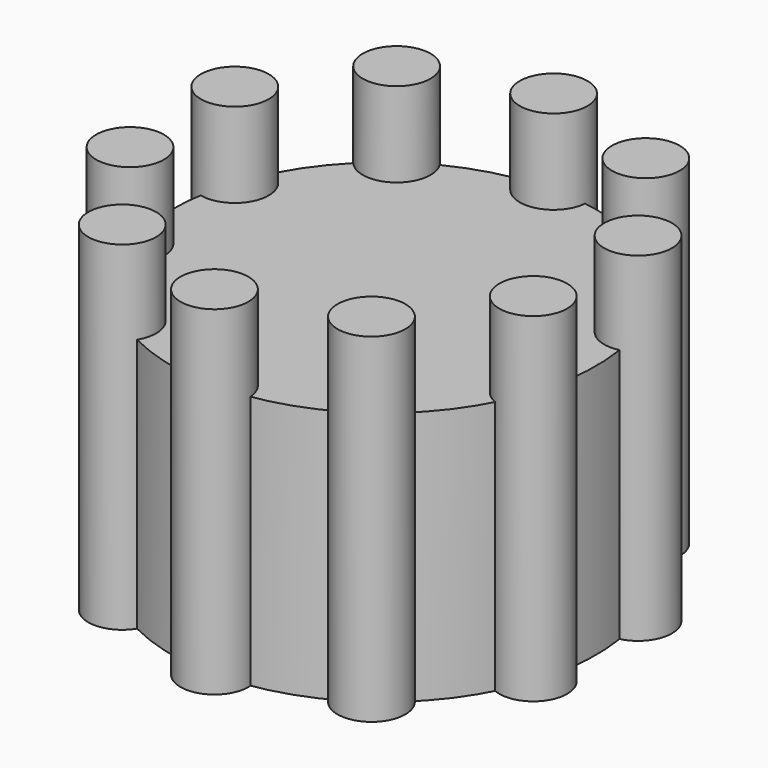
from build123d import *

# Parameters (mm, degrees)
F0_R     = 31.75
F1_DEPTH = 38.1
F2_R     = 5.08
F3_DEPTH = 50.8


with BuildPart() as f1:
    # F0 (on Top) → F1 (new body)
    with BuildSketch(Plane.XY):
        Circle(F0_R)
    extrude(amount=F1_DEPTH)

    # F2 (on Top) → F3, piece 2 (join)
    with BuildSketch(Plane.XY):
        with Locations((-18.6621817603, 25.6862895714)):
            Circle(F2_R)
    extrude(amount=F3_DEPTH)


with BuildPart() as f3:
    # F2 (on Top) → F3 (new body)
    with BuildSketch(Plane.XY):
        with Locations((0, 31.75)):
            Circle(F2_R)
    extrude(amount=F3_DEPTH)


with BuildPart() as f3b:
    # F2 (on Top) → F3, piece 3 (new body)
    with BuildSketch(Plane.XY):
        with Locations((-30.1960443924, 9.8112895714)):
            Circle(F2_R)
    extrude(amount=F3_DEPTH)


with BuildPart() as f3c:
    # F2 (on Top) → F3, piece 4 (new body)
    with BuildSketch(Plane.XY):
        with Locations((-30.1960443924, -9.8112895714)):
            Circle(F2_R)
    extrude(amount=F3_DEPTH)


with BuildPart() as f3d:
    # F2 (on Top) → F3, piece 5 (new body)
    with BuildSketch(Plane.XY):
        with Locations((-18.6621817603, -25.6862895714)):
            Circle(F2_R)
    extrude(amount=F3_DEPTH)


with BuildPart() as f3e:
    # F2 (on Top) → F3, piece 6 (new body)
    with BuildSketch(Plane.XY):
        with Locations((0, -31.75)):
            Circle(F2_R)
    extrude(amount=F3_DEPTH)


with BuildPart() as f3f:
    # F2 (on Top) → F3, piece 7 (new body)
    with BuildSketch(Plane.XY):
        with Locations((18.6621817603, -25.6862895714)):
            Circle(F2_R)
    extrude(amount=F3_DEPTH)


with BuildPart() as f3g:
    # F2 (on Top) → F3, piece 8 (new body)
    with BuildSketch(Plane.XY):
        with Locations((30.1960443924, -9.8112895714)):
            Circle(F2_R)
    extrude(amount=F3_DEPTH)


with BuildPart() as f3h:
    # F2 (on Top) → F3, piece 9 (new body)
    with BuildSketch(Plane.XY):
        with Locations((30.1960443924, 9.8112895714)):
            Circle(F2_R)
    extrude(amount=F3_DEPTH)


with BuildPart() as f3i:
    # F2 (on Top) → F3, piece 10 (new body)
    with BuildSketch(Plane.XY):
        with Locations((18.6621817603, 25.6862895714)):
            Circle(F2_R)
    extrude(amount=F3_DEPTH)


solid = Compound([f1.part, f3.part, f3b.part, f3c.part, f3d.part, f3e.part, f3f.part, f3g.part, f3h.part, f3i.part])
